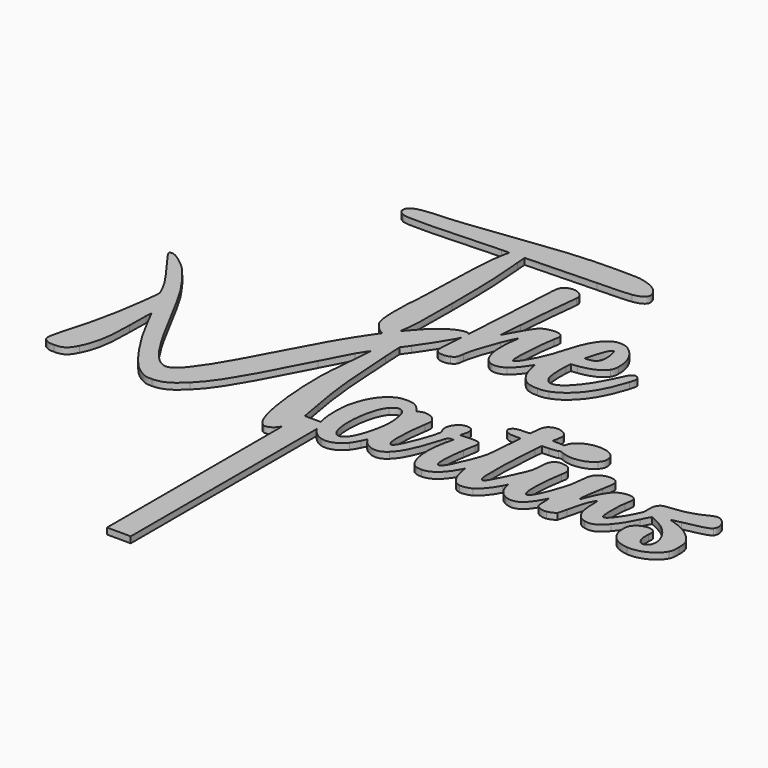
from build123d import *

# Parameters (mm, degrees)
F1_DEPTH = 1.524


# Not quite as in the source:
# - ends of sketch curves that miss each other by under 0.0002 mm in the source are joined


with BuildPart() as f1:
    # F0 (on Top) → F1 (new body)
    with BuildSketch(Plane.XY):
        with BuildLine():
            add(Edge.make_bspline(
                [(-16.4951387862, 3474.825739188), (-16.6800585023, 3474.8804924692), (-16.8650518694, 3474.9520282822), (-17.0115018566, 3475.0294197741)],
                knots=[0.5346499123, 0.5346499123, 0.5346499123, 0.5346499123, 1, 1, 1, 1], degree=3))
            add(Edge.make_bspline(
                [(-16.4951387862, 3474.825739188), (-15.7866961372, 3475.8123794255), (-15.094304248, 3476.7288703178), (-14.4178850512, 3477.5752871703)],
                knots=[0.0597909067, 0.0597909067, 0.0597909067, 0.0597909067, 0.2184884646, 0.2184884646, 0.2184884646, 0.2184884646], degree=3))
            add(Edge.make_bspline(
                [(-14.4058442585, 3477.6385135946), (-14.4097287654, 3477.6176536184), (-14.4137442865, 3477.5965715564), (-14.4178850512, 3477.5752871703)],
                knots=[0, 0, 0, 0, 0.0299805495, 0.0299805495, 0.0299805495, 0.0299805495], degree=3))
            add(Edge.make_bspline(
                [(-13.764209968, 3492.7401815257), (-13.7508003194, 3482.6742635991), (-13.8343750054, 3480.7073148376), (-14.4058442585, 3477.6385135946)],
                knots=[0, 0, 0, 0, 1, 1, 1, 1], degree=3))
            add(Edge.make_bspline(
                [(-14.5580975351, 3513.8236564948), (-13.9877605118, 3508.4516247626), (-13.7777050082, 3502.8731476952), (-13.764209968, 3492.7401815257)],
                knots=[0, 0, 0, 0, 1, 1, 1, 1], degree=3))
            add(Edge.make_bspline(
                [(-14.7308827548, 3516.2445566504), (-14.7727673494, 3516.2026736371), (-14.6950135262, 3515.1132677764), (-14.5580975351, 3513.8236564948)],
                knots=[0, 0, 0, 0, 1, 1, 1, 1], degree=3))
            add(Edge.make_bspline(
                [(2.5366157885, 3516.7758823493), (-6.7649300297, 3516.5842746005), (-14.6332769589, 3516.3421640277), (-14.7308827548, 3516.2445566504)],
                knots=[0, 0, 0, 0, 1, 1, 1, 1], degree=3))
            add(Edge.make_bspline(
                [(10.9317057324, 3517.1545373014), (10.1299399967, 3516.9908842422), (7.7392827101, 3516.8830551705), (2.5366157885, 3516.7758823493)],
                knots=[0, 0, 0, 0, 1, 1, 1, 1], degree=3))
            add(Edge.make_bspline(
                [(13.5480783988, 3520.1762023646), (14.3093700831, 3518.5046279958), (13.614522575, 3517.7021443379), (10.9317057324, 3517.1545373014)],
                knots=[0, 0, 0, 0, 1, 1, 1, 1], degree=3))
            add(Edge.make_bspline(
                [(8.6247227555, 3523.207953128), (11.0429694452, 3522.689428267), (12.9337378033, 3521.525111808), (13.5480783988, 3520.1762023646)],
                knots=[0, 0, 0, 0, 1, 1, 1, 1], degree=3))
            add(Edge.make_bspline(
                [(2.062217843, 3523.496576838), (6.5131268977, 3523.4962605727), (7.4782768672, 3523.4537782367), (8.6247227555, 3523.207953128)],
                knots=[0, 0, 0, 0, 1, 1, 1, 1], degree=3))
            add(Edge.make_bspline(
                [(-23.2390059159, 3521.3613464746), (-10.9639432633, 3523.0044806865), (-5.1261808362, 3523.4971429529), (2.062217843, 3523.496576838)],
                knots=[0, 0, 0, 0, 1, 1, 1, 1], degree=3))
            add(Edge.make_bspline(
                [(-37.4580975839, 3519.7783675035), (-36.0309520126, 3519.7811664514), (-30.1663086165, 3520.4340597865), (-23.2390059159, 3521.3613464746)],
                knots=[0, 0, 0, 0, 1, 1, 1, 1], degree=3))
            add(Edge.make_bspline(
                [(-43.4768191074, 3519.1378195843), (-42.3460378392, 3519.487082421), (-39.6493843899, 3519.7740757834), (-37.4580975839, 3519.7783675035)],
                knots=[0, 0, 0, 0, 1, 1, 1, 1], degree=3))
            add(Edge.make_bspline(
                [(-45.4566430292, 3517.290477614), (-45.4566430292, 3518.1528603379), (-44.8583655482, 3518.7111033763), (-43.4768191074, 3519.1378195843)],
                knots=[0, 0, 0, 0, 1, 1, 1, 1], degree=3))
            add(Edge.make_bspline(
                [(-44.1915818412, 3515.7274518205), (-45.1570717959, 3516.2424645554), (-45.4566430292, 3516.6125961578), (-45.4566430292, 3517.290477614)],
                knots=[0, 0, 0, 0, 1, 1, 1, 1], degree=3))
            add(Edge.make_bspline(
                [(-20.2740187566, 3516.06545245), (-37.5407345433, 3515.2545118581), (-43.1561956746, 3515.1751545697), (-44.1915818412, 3515.7274518205)],
                knots=[0, 0, 0, 0, 1, 1, 1, 1], degree=3))
            add(Edge.make_bspline(
                [(-18.4159601368, 3516.0222648424), (-18.4159601368, 3516.094014369), (-19.2520865158, 3516.1134488715), (-20.2740187566, 3516.06545245)],
                knots=[0, 0, 0, 0, 1, 1, 1, 1], degree=3))
            add(Edge.make_bspline(
                [(-18.7238728673, 3514.4760232482), (-18.5545207074, 3515.2547079426), (-18.4159601368, 3515.9505168971), (-18.4159601368, 3516.0222648424)],
                knots=[0, 0, 0, 0, 1, 1, 1, 1], degree=3))
            add(Edge.make_bspline(
                [(-19.8305136054, 3497.1663617968), (-19.6046068851, 3507.2168934167), (-19.3139859597, 3511.7626535966), (-18.7238728673, 3514.4760232482)],
                knots=[0, 0, 0, 0, 1, 1, 1, 1], degree=3))
            add(Edge.make_bspline(
                [(-20.0594944244, 3490.3666579116), (-20.0147033517, 3490.4962634303), (-19.9116625366, 3493.5561301787), (-19.8305136054, 3497.1663617968)],
                knots=[0, 0, 0, 0, 1, 1, 1, 1], degree=3))
            add(Edge.make_bspline(
                [(-20.3144422056, 3486.8892735315), (-20.2190123149, 3488.6722191432), (-20.1042870784, 3490.2370365797), (-20.0594944244, 3490.3666579116)],
                knots=[0, 0, 0, 0, 1, 1, 1, 1], degree=3))
            add(Edge.make_bspline(
                [(-19.8302368732, 3478.1253882061), (-20.3470112059, 3479.5065820111), (-20.5311772323, 3482.8399075484), (-20.3144422056, 3486.8892735315)],
                knots=[0, 0, 0, 0, 1, 1, 1, 1], degree=3))
            add(Edge.make_bspline(
                [(-17.0115018566, 3475.0294197741), (-18.0581945076, 3475.5825677785), (-19.4513605354, 3477.1127383516), (-19.8302368732, 3478.1253882061)],
                knots=[0, 0, 0, 0, 1, 1, 1, 1], degree=3))
        make_face()
        with BuildLine():
            Line((-56.2574582039, 3453.6457123253), (-54.4877957346, 3450.1823891003))
            add(Edge.make_bspline(
                [(-48.7301844216, 3440.3937599355), (-50.9593487409, 3443.67603551), (-52.5123046474, 3446.3162466731), (-54.4877957346, 3450.1823891003)],
                knots=[0, 0, 0, 0, 1, 1, 1, 1], degree=3))
            add(Edge.make_bspline(
                [(-41.7754741704, 3432.9327184318), (-43.9459380692, 3434.0343890607), (-45.6602446236, 3435.8735049705), (-48.7301844216, 3440.3937599355)],
                knots=[0, 0, 0, 0, 1, 1, 1, 1], degree=3))
            add(Edge.make_bspline(
                [(-39.1483073695, 3432.3396798854), (-40.5110945342, 3432.3295435827), (-40.6480516397, 3432.3604680034), (-41.7754741704, 3432.9327184318)],
                knots=[0, 0, 0, 0, 1, 1, 1, 1], degree=3))
            add(Edge.make_bspline(
                [(-32.502838163, 3435.8000523553), (-35.077889187, 3433.233766624), (-36.7608649197, 3432.3574207873), (-39.1483073695, 3432.3396798854)],
                knots=[0, 0, 0, 0, 1, 1, 1, 1], degree=3))
            add(Edge.make_bspline(
                [(-18.9330217551, 3458.1046165667), (-26.3784697984, 3443.5673335461), (-28.94959597, 3439.3412005633), (-32.502838163, 3435.8000523553)],
                knots=[0, 0, 0, 0, 1, 1, 1, 1], degree=3))
            add(Edge.make_bspline(
                [(-15.3817451509, 3464.910389583), (-15.6422655267, 3464.4721866194), (-17.2403414217, 3461.4095889202), (-18.9330217551, 3458.1046165667)],
                knots=[0, 0, 0, 0, 1, 1, 1, 1], degree=3))
            add(Edge.make_bspline(
                [(-13.6368019773, 3467.5135091521), (-13.722075008, 3467.5135091521), (-14.7129752979, 3466.0352772473), (-15.3817451509, 3464.910389583)],
                knots=[0, 0, 0, 0, 1, 1, 1, 1], degree=3))
            add(Edge.make_bspline(
                [(-14.1663692412, 3460.3975399699), (-13.7542202128, 3464.3164749818), (-13.5162985738, 3467.5135091521), (-13.6368019773, 3467.5135091521)],
                knots=[0, 0, 0, 0, 1, 1, 1, 1], degree=3))
            add(Edge.make_bspline(
                [(-14.5609813588, 3447.9841270632), (-14.7854601413, 3452.0795128096), (-14.6746866397, 3455.5641855235), (-14.1663692412, 3460.3975399699)],
                knots=[0, 0, 0, 0, 1, 1, 1, 1], degree=3))
            add(Edge.make_bspline(
                [(-11.0901911101, 3431.1923010145), (-12.8122066311, 3432.9143165355), (-14.0679759446, 3438.9897792159), (-14.5609813588, 3447.9841270632)],
                knots=[0, 0, 0, 0, 1, 1, 1, 1], degree=3))
            add(Edge.make_bspline(
                [(-10.2336814328, 3430.6335930661), (-10.4286321059, 3430.6647531045), (-10.8140614606, 3430.916171365), (-11.0901911101, 3431.1923010145)],
                knots=[0, 0, 0, 0, 1, 1, 1, 1], degree=3))
            add(Edge.make_bspline(
                [(-7.840324822, 3431.8184825826), (-8.489377115, 3430.9675296866), (-9.4249847431, 3430.5043354393), (-10.2336814328, 3430.6335930661)],
                knots=[0, 0, 0, 0, 1, 1, 1, 1], degree=3))
            add(Edge.make_bspline(
                [(-7.3343984416, 3432.5808147994), (-7.4816183586, 3432.321105511), (-7.6498403129, 3432.0682205632), (-7.840324822, 3431.8184825826)],
                knots=[0.7774513502, 0.7774513502, 0.7774513502, 0.7774513502, 1, 1, 1, 1], degree=3))
            Line((-7.3343984416, 3432.5808147994), (-7.3343984416, 3438.6502356796))
            Line((-7.3343984416, 3438.6502356796), (-6.6488588735, 3438.6502356796))
            add(Edge.make_bspline(
                [(-7.5903503126, 3443.9517445266), (-7.1005108992, 3441.4777591259), (-6.8078684627, 3439.8717466959), (-6.6488588735, 3438.6502356796)],
                knots=[0, 0, 0, 0, 0.5048196065, 0.5048196065, 0.5048196065, 0.5048196065], degree=3))
            add(Edge.make_bspline(
                [(-10.0368094481, 3467.7243205298), (-9.4481780587, 3456.3496999669), (-8.8021318672, 3450.0719824664), (-7.5903503126, 3443.9517445266)],
                knots=[0, 0, 0, 0, 1, 1, 1, 1], degree=3))
            Line((-10.0368094481, 3467.7243205298), (-10.2727591729, 3472.2837781597))
            Line((-10.2727591729, 3472.2837781597), (-8.8698205474, 3474.2172534022))
            add(Edge.make_bspline(
                [(-3.8857119219, 3482.0310698688), (-4.5791504681, 3480.6626342059), (-7.3860524187, 3476.2621251889), (-8.8698205474, 3474.2172534022)],
                knots=[0, 0, 0, 0, 1, 1, 1, 1], degree=3))
            add(Edge.make_bspline(
                [(-3.5395519409, 3482.8531070297), (-3.6464231613, 3482.5565940157), (-3.7706794884, 3482.2580737216), (-3.8857119219, 3482.0310698688)],
                knots=[0.4932655399, 0.4932655399, 0.4932655399, 0.4932655399, 1, 1, 1, 1], degree=3))
            add(Edge.make_bspline(
                [(-3.5395519361, 3482.8531070287), (-3.4918571938, 3483.5093905716), (-3.4436011891, 3484.1852250498), (-3.3951575292, 3484.8747923712)],
                knots=[0.121112451, 0.121112451, 0.121112451, 0.121112451, 0.2158785304, 0.2158785304, 0.2158785304, 0.2158785304], degree=3))
            add(Edge.make_bspline(
                [(-5.5774766672, 3484.9908022801), (-4.4187556834, 3485.3423771205), (-3.6978778733, 3485.3075858697), (-3.3951575098, 3484.8747923775)],
                knots=[0, 0, 0, 0, 0.6224653627, 0.6224653627, 0.6224653627, 0.6224653627], degree=3))
            add(Edge.make_bspline(
                [(-14.4178850512, 3477.5752871703), (-11.0868356496, 3481.7434958245), (-8.1431405884, 3484.2123364092), (-5.5774766672, 3484.9908022801)],
                knots=[0.2184884646, 0.2184884646, 0.2184884646, 0.2184884646, 1, 1, 1, 1], degree=3))
            add(Edge.make_bspline(
                [(-14.4178850512, 3477.5752871703), (-14.5518593236, 3476.8866317296), (-14.8169440207, 3475.9861746652), (-15.0176831954, 3475.5432560021)],
                knots=[0.0299805495, 0.0299805495, 0.0299805495, 0.0299805495, 1, 1, 1, 1], degree=3))
            add(Edge.make_bspline(
                [(-15.0176831954, 3475.5432560021), (-15.3628867671, 3474.7815942874), (-15.4370841871, 3474.7136446883), (-15.916623025, 3474.7200490606)],
                knots=[0, 0, 0, 0, 1, 1, 1, 1], degree=3))
            add(Edge.make_bspline(
                [(-15.916623025, 3474.7200490606), (-16.0703201742, 3474.7220781551), (-16.2826808699, 3474.7628320611), (-16.4951387862, 3474.825739188)],
                knots=[0, 0, 0, 0, 0.5346499123, 0.5346499123, 0.5346499123, 0.5346499123], degree=3))
            add(Edge.make_bspline(
                [(-17.3027168449, 3473.6806824433), (-17.0312429994, 3474.0723282808), (-16.7620517048, 3474.4540125199), (-16.4951387862, 3474.825739188)],
                knots=[0, 0, 0, 0, 0.0597909067, 0.0597909067, 0.0597909067, 0.0597909067], degree=3))
            add(Edge.make_bspline(
                [(-27.1440658534, 3456.8697112749), (-22.5396368796, 3465.6083143524), (-20.5916703611, 3468.9358253523), (-17.3027168449, 3473.6806824433)],
                knots=[0, 0, 0, 0, 1, 1, 1, 1], degree=3))
            add(Edge.make_bspline(
                [(-36.4910811334, 3441.0044792933), (-34.0927812959, 3444.0904363473), (-32.0556058252, 3447.5482518122), (-27.1440658534, 3456.8697112749)],
                knots=[0, 0, 0, 0, 1, 1, 1, 1], degree=3))
            add(Edge.make_bspline(
                [(-40.369586371, 3438.1043091253), (-39.1970723156, 3438.096228547), (-38.1327937328, 3438.8920437511), (-36.4910811334, 3441.0044792933)],
                knots=[0, 0, 0, 0, 1, 1, 1, 1], degree=3))
            add(Edge.make_bspline(
                [(-47.3935397464, 3445.5162630923), (-44.7686611249, 3440.8615732375), (-42.1674834247, 3438.116706725), (-40.369586371, 3438.1043091253)],
                knots=[0, 0, 0, 0, 1, 1, 1, 1], degree=3))
            add(Edge.make_bspline(
                [(-48.7851940261, 3447.9160256568), (-48.5890241503, 3447.6055891292), (-47.9627809104, 3446.5256965287), (-47.3935397464, 3445.5162630923)],
                knots=[0, 0, 0, 0, 1, 1, 1, 1], degree=3))
            add(Edge.make_bspline(
                [(-51.6322332055, 3453.2134693813), (-50.2625309, 3450.6103118604), (-48.9813623205, 3448.2264621843), (-48.7851940261, 3447.9160256568)],
                knots=[0, 0, 0, 0, 1, 1, 1, 1], degree=3))
            add(Edge.make_bspline(
                [(-57.8490759616, 3464.4830187058), (-56.3952502498, 3462.1380902186), (-54.9414213754, 3459.5026688934), (-51.6322332055, 3453.2134693813)],
                knots=[0, 0, 0, 0, 1, 1, 1, 1], degree=3))
            add(Edge.make_bspline(
                [(-63.0135538486, 3471.4352652504), (-61.5574700026, 3469.8649811683), (-59.3104436124, 3466.8401107564), (-57.8490759616, 3464.4830187058)],
                knots=[0, 0, 0, 0, 1, 1, 1, 1], degree=3))
            add(Edge.make_bspline(
                [(-68.7254664075, 3475.5782742252), (-67.7419287737, 3475.5782742252), (-65.0339055869, 3473.6140706465), (-63.0135538486, 3471.4352652504)],
                knots=[0, 0, 0, 0, 1, 1, 1, 1], degree=3))
            add(Edge.make_bspline(
                [(-66.2668437086, 3470.7744431443), (-69.7205508873, 3475.3821802531), (-69.8209129353, 3475.5782742252), (-68.7254664075, 3475.5782742252)],
                knots=[0, 0, 0, 0, 1, 1, 1, 1], degree=3))
            add(Edge.make_bspline(
                [(-60.9473141901, 3462.7309152858), (-61.9172707991, 3464.737201125), (-63.2340208058, 3466.7282271636), (-66.2668437086, 3470.7744431443)],
                knots=[0, 0, 0, 0, 1, 1, 1, 1], degree=3))
            add(Edge.make_bspline(
                [(-60.330889604, 3459.7650093759), (-60.1653972644, 3461.0192163389), (-60.1997966501, 3461.1847274567), (-60.9473141901, 3462.7309152858)],
                knots=[0, 0, 0, 0, 1, 1, 1, 1], degree=3))
            add(Edge.make_bspline(
                [(-60.7262975243, 3456.4219918885), (-60.5604653971, 3457.86927249), (-60.3825319714, 3459.3736310709), (-60.330889604, 3459.7650093759)],
                knots=[0, 0, 0, 0, 1, 1, 1, 1], degree=3))
            add(Edge.make_bspline(
                [(-64.6322818676, 3437.7794682948), (-62.743153345, 3444.1123551137), (-61.4048953214, 3450.4996063558), (-60.7262975243, 3456.4219918885)],
                knots=[0, 0, 0, 0, 1, 1, 1, 1], degree=3))
            add(Edge.make_bspline(
                [(-65.4686612587, 3434.4119339216), (-65.3597394904, 3435.0871366108), (-64.9833695551, 3436.6025265252), (-64.6322818676, 3437.7794682948)],
                knots=[0, 0, 0, 0, 1, 1, 1, 1], degree=3))
            add(Edge.make_bspline(
                [(-64.6167247776, 3432.0724293842), (-65.5929930536, 3432.6318299535), (-65.7058349302, 3432.9417051102), (-65.4686612587, 3434.4119339216)],
                knots=[0, 0, 0, 0, 1, 1, 1, 1], degree=3))
            add(Edge.make_bspline(
                [(-62.616462211, 3431.6983618602), (-63.7444982964, 3431.6967647204), (-64.066075269, 3431.7569073106), (-64.6167247776, 3432.0724293842)],
                knots=[0, 0, 0, 0, 1, 1, 1, 1], degree=3))
            add(Edge.make_bspline(
                [(-58.5744363502, 3434.4829354808), (-59.6836665104, 3432.2802979133), (-60.5241049689, 3431.7013157781), (-62.616462211, 3431.6983618602)],
                knots=[0, 0, 0, 0, 1, 1, 1, 1], degree=3))
            add(Edge.make_bspline(
                [(-56.4171073445, 3447.0353311722), (-56.3913222348, 3441.1183553574), (-56.9915006679, 3437.6262251078), (-58.5744363502, 3434.4829354808)],
                knots=[0, 0, 0, 0, 1, 1, 1, 1], degree=3))
            add(Edge.make_bspline(
                [(-56.3445197148, 3452.000914558), (-56.3924022808, 3451.0962756278), (-56.425067742, 3448.8617632623), (-56.4171073445, 3447.0353311722)],
                knots=[0, 0, 0, 0, 1, 1, 1, 1], degree=3))
            Line((-56.3445197148, 3452.000914558), (-56.2574582039, 3453.6457123253))
        make_face()
        with BuildLine():
            add(Edge.make_bspline(
                [(-3.301422855, 3483.6454808665), (-3.3479639421, 3483.4284685297), (-3.4355213403, 3483.1417387756), (-3.5395519409, 3482.8531070297)],
                knots=[0, 0, 0, 0, 0.4932655399, 0.4932655399, 0.4932655399, 0.4932655399], degree=3))
            add(Edge.make_bspline(
                [(-3.7188856562, 3480.4448304544), (-3.660544386, 3481.2075598501), (-3.6005065222, 3482.0143669549), (-3.5395519409, 3482.8531070297)],
                knots=[0, 0, 0, 0, 0.121112451, 0.121112451, 0.121112451, 0.121112451], degree=3))
            add(Edge.make_bspline(
                [(-3.1856006938, 3475.3377309988), (-4.0624019525, 3475.8723458569), (-4.0659994703, 3475.906802961), (-3.7188856562, 3480.4448304544)],
                knots=[0, 0, 0, 0, 1, 1, 1, 1], degree=3))
            add(Edge.make_bspline(
                [(-0.2639387175, 3475.3287648777), (-1.0620152186, 3474.9214468017), (-2.5101702936, 3474.9258903291), (-3.1856006938, 3475.3377309988)],
                knots=[0, 0, 0, 0, 1, 1, 1, 1], degree=3))
            add(Edge.make_bspline(
                [(1.0625617483, 3477.6703456968), (0.8960101176, 3476.1384356645), (0.7225623221, 3475.8322592305), (-0.2639387175, 3475.3287648777)],
                knots=[0, 0, 0, 0, 1, 1, 1, 1], degree=3))
            add(Edge.make_bspline(
                [(3.5972320192, 3485.9404776405), (2.2704516585, 3482.5973320657), (1.2286753516, 3479.1982233465), (1.0625617483, 3477.6703456968)],
                knots=[0, 0, 0, 0, 1, 1, 1, 1], degree=3))
            add(Edge.make_bspline(
                [(5.2550361969, 3489.3628792988), (5.1405260208, 3489.4773989628), (4.3679057135, 3487.8823781905), (3.5972320192, 3485.9404776405)],
                knots=[0, 0, 0, 0, 1, 1, 1, 1], degree=3))
            add(Edge.make_bspline(
                [(5.0713414058, 3487.9181794221), (5.2043325445, 3488.680805746), (5.2869948052, 3489.3309206905), (5.2550361969, 3489.3628792988)],
                knots=[0, 0, 0, 0, 1, 1, 1, 1], degree=3))
            add(Edge.make_bspline(
                [(4.983539834, 3482.1273460211), (4.7530709868, 3483.4020691138), (4.7977576919, 3486.3493454164), (5.0713414058, 3487.9181794221)],
                knots=[0, 0, 0, 0, 1, 1, 1, 1], degree=3))
            add(Edge.make_bspline(
                [(7.6110814093, 3477.9409422849), (6.2673666234, 3478.4541143558), (5.3969112278, 3479.8410009361), (4.983539834, 3482.1273460211)],
                knots=[0, 0, 0, 0, 1, 1, 1, 1], degree=3))
            add(Edge.make_bspline(
                [(11.0315064095, 3478.5305714913), (9.9027539832, 3477.8062607081), (8.5667940223, 3477.5759563189), (7.6110814093, 3477.9409422849)],
                knots=[0, 0, 0, 0, 1, 1, 1, 1], degree=3))
            add(Edge.make_bspline(
                [(14.1259899759, 3482.1316788556), (13.3519701947, 3480.814212508), (11.8298153655, 3479.0428422061), (11.0315064095, 3478.5305714913)],
                knots=[0, 0, 0, 0, 1, 1, 1, 1], degree=3))
            Line((14.1259899759, 3482.1316788556), (14.5360516534, 3482.8296447396))
            Line((14.5360516534, 3482.8296447396), (14.8073092359, 3481.5782145859))
            add(Edge.make_bspline(
                [(16.4588181529, 3477.5675278487), (15.662568084, 3478.6491709777), (15.1972738351, 3479.7791236307), (14.8073092359, 3481.5782145859)],
                knots=[0, 0, 0, 0, 1, 1, 1, 1], degree=3))
            add(Edge.make_bspline(
                [(21.0381356622, 3475.4371964347), (18.8022839132, 3475.4327687206), (17.6283023868, 3475.9788956354), (16.4588181529, 3477.5675278487)],
                knots=[0, 0, 0, 0, 1, 1, 1, 1], degree=3))
            add(Edge.make_bspline(
                [(23.5682580381, 3475.8376989936), (22.6999658971, 3475.5257507179), (22.154511046, 3475.4394102918), (21.0381356622, 3475.4371964347)],
                knots=[0, 0, 0, 0, 1, 1, 1, 1], degree=3))
            add(Edge.make_bspline(
                [(33.1572652914, 3488.5029855828), (31.1569584476, 3481.8590265431), (27.7301796776, 3477.3329064381), (23.5682580381, 3475.8376989936)],
                knots=[0, 0, 0, 0, 1, 1, 1, 1], degree=3))
            add(Edge.make_bspline(
                [(32.8994885171, 3491.1109724748), (33.651032905, 3490.7525806403), (33.6963916739, 3490.2936638811), (33.1572652914, 3488.5029855828)],
                knots=[0, 0, 0, 0, 1, 1, 1, 1], degree=3))
            add(Edge.make_bspline(
                [(31.9313624912, 3491.1365108975), (32.3257010394, 3491.3252264003), (32.4574777193, 3491.321747482), (32.8994885171, 3491.1109724748)],
                knots=[0, 0, 0, 0, 1, 1, 1, 1], degree=3))
            add(Edge.make_bspline(
                [(31.2100261831, 3490.3664048994), (31.3557011416, 3490.669814012), (31.6803031918, 3491.0163775245), (31.9313624912, 3491.1365108975)],
                knots=[0, 0, 0, 0, 1, 1, 1, 1], degree=3))
            add(Edge.make_bspline(
                [(29.8435988048, 3487.5218041254), (30.449457165, 3488.7829119972), (31.0643496434, 3490.0629799735), (31.2100261831, 3490.3664048994)],
                knots=[0, 0, 0, 0, 1, 1, 1, 1], degree=3))
            add(Edge.make_bspline(
                [(25.2460517639, 3480.5527718002), (26.7766540392, 3482.0754943256), (28.4340344214, 3484.5877793388), (29.8435988048, 3487.5218041254)],
                knots=[0, 0, 0, 0, 1, 1, 1, 1], degree=3))
            add(Edge.make_bspline(
                [(21.9211926485, 3478.6663758098), (22.9317820345, 3478.6663758098), (23.9048180792, 3479.2184485122), (25.2460517639, 3480.5527718002)],
                knots=[0, 0, 0, 0, 1, 1, 1, 1], degree=3))
            add(Edge.make_bspline(
                [(19.9306331012, 3480.5723011823), (20.3094635806, 3479.3572099113), (21.0309675092, 3478.6663758098), (21.9211926485, 3478.6663758098)],
                knots=[0, 0, 0, 0, 1, 1, 1, 1], degree=3))
            add(Edge.make_bspline(
                [(19.6069687776, 3485.9779392649), (19.4547661034, 3484.1507797647), (19.6068454341, 3481.6108531646), (19.9306331012, 3480.5723011823)],
                knots=[0, 0, 0, 0, 1, 1, 1, 1], degree=3))
            Line((19.6069687776, 3485.9779392649), (19.7181075656, 3487.3121676733))
            Line((19.7181075656, 3487.3121676733), (21.2162325575, 3487.5081572779))
            add(Edge.make_bspline(
                [(27.0846142094, 3490.238254201), (26.1960020232, 3488.8955024429), (23.9954865958, 3487.8717833031), (21.2162325575, 3487.5081572779)],
                knots=[0, 0, 0, 0, 1, 1, 1, 1], degree=3))
            add(Edge.make_bspline(
                [(27.5768590056, 3492.113754852), (27.5310527213, 3491.1068768392), (27.4466620708, 3490.7853299118), (27.0846142094, 3490.238254201)],
                knots=[0, 0, 0, 0, 1, 1, 1, 1], degree=3))
            add(Edge.make_bspline(
                [(25.0059494757, 3498.5539916006), (26.7593021436, 3496.9138081439), (27.6892486229, 3494.5842612194), (27.5768590056, 3492.113754852)],
                knots=[0, 0, 0, 0, 1, 1, 1, 1], degree=3))
            add(Edge.make_bspline(
                [(21.6820296683, 3500.0108202514), (22.9531331047, 3500.0163548941), (23.8743142913, 3499.6125789894), (25.0059494757, 3498.5539916006)],
                knots=[0, 0, 0, 0, 1, 1, 1, 1], degree=3))
            add(Edge.make_bspline(
                [(15.1826845169, 3491.237921365), (16.6399654271, 3496.8318479922), (18.9864388703, 3499.9991500619), (21.6820296683, 3500.0108202514)],
                knots=[0, 0, 0, 0, 1, 1, 1, 1], degree=3))
            add(Edge.make_bspline(
                [(11.5406682364, 3482.749424047), (13.07443949, 3485.1272804956), (14.3889060613, 3488.1909266143), (15.1826845169, 3491.237921365)],
                knots=[0, 0, 0, 0, 1, 1, 1, 1], degree=3))
            add(Edge.make_bspline(
                [(10.0721425137, 3481.5517906203), (10.3716742138, 3481.2522715708), (10.8005979535, 3481.6020609893), (11.5406682364, 3482.749424047)],
                knots=[0, 0, 0, 0, 1, 1, 1, 1], degree=3))
            add(Edge.make_bspline(
                [(10.7689540292, 3493.3322934147), (10.0735309183, 3490.1320523143), (9.5942767192, 3482.0296674841), (10.0721425137, 3481.5517906203)],
                knots=[0, 0, 0, 0, 1, 1, 1, 1], degree=3))
            add(Edge.make_bspline(
                [(10.4849066781, 3495.6397650215), (11.0271419484, 3495.2367165271), (11.0834276833, 3494.7794601607), (10.7689540292, 3493.3322934147)],
                knots=[0, 0, 0, 0, 1, 1, 1, 1], degree=3))
            add(Edge.make_bspline(
                [(5.9370132887, 3495.1916487222), (7.1459864076, 3496.0835959261), (9.5668834005, 3496.3221390263), (10.4849066781, 3495.6397650215)],
                knots=[0, 0, 0, 0, 1, 1, 1, 1], degree=3))
            add(Edge.make_bspline(
                [(2.4248175873, 3489.8147275286), (4.1401156334, 3493.0214678808), (5.2048101051, 3494.6514359685), (5.9370132887, 3495.1916487222)],
                knots=[0, 0, 0, 0, 1, 1, 1, 1], degree=3))
            Line((2.4248175873, 3489.8147275286), (1.6635464602, 3488.3915336921))
            Line((1.6635464602, 3488.3915336921), (1.7489728796, 3489.4193959074))
            add(Edge.make_bspline(
                [(2.0702256803, 3493.9261763894), (1.9405221194, 3492.0127713426), (1.7959572521, 3489.9847201257), (1.7489728796, 3489.4193959074)],
                knots=[0, 0, 0, 0, 1, 1, 1, 1], degree=3))
            add(Edge.make_bspline(
                [(3.5023729873, 3509.3441096175), (3.0602325208, 3505.8495520317), (2.3876390203, 3498.6086738705), (2.0702256803, 3493.9261763894)],
                knots=[0, 0, 0, 0, 1, 1, 1, 1], degree=3))
            add(Edge.make_bspline(
                [(2.146034472, 3511.5184335343), (3.1461823592, 3511.0131839091), (3.6178746551, 3510.2570252105), (3.5023729873, 3509.3441096175)],
                knots=[0, 0, 0, 0, 1, 1, 1, 1], degree=3))
            add(Edge.make_bspline(
                [(-1.5014105023, 3510.7593810082), (-0.7438665617, 3511.8232500275), (0.8755524969, 3512.160262328), (2.146034472, 3511.5184335343)],
                knots=[0, 0, 0, 0, 1, 1, 1, 1], degree=3))
            add(Edge.make_bspline(
                [(-2.365749327, 3501.5165435171), (-1.9443969785, 3509.9288208985), (-1.9219563743, 3510.1687871926), (-1.5014105023, 3510.7593810082)],
                knots=[0, 0, 0, 0, 1, 1, 1, 1], degree=3))
            add(Edge.make_bspline(
                [(-3.3951575292, 3484.8747923712), (-2.9943209219, 3490.5804683344), (-2.5806367367, 3497.2263466322), (-2.365749327, 3501.5165435171)],
                knots=[0.2158785304, 0.2158785304, 0.2158785304, 0.2158785304, 1, 1, 1, 1], degree=3))
            add(Edge.make_bspline(
                [(-3.3951575292, 3484.8747923712), (-3.2115530404, 3484.6122965925), (-3.1817722025, 3484.2033914808), (-3.301422855, 3483.6454808665)],
                knots=[0.6224653627, 0.6224653627, 0.6224653627, 0.6224653627, 1, 1, 1, 1], degree=3))
        make_face()
        with BuildLine():
            Line((20.3089528121, 3490.7965415165), (20.4186873822, 3491.2544304135))
            add(Edge.make_bspline(
                [(22.7127572471, 3496.693497738), (22.1171949037, 3496.693497738), (21.202353255, 3494.5244870782), (20.4186873822, 3491.2544304135)],
                knots=[0, 0, 0, 0, 1, 1, 1, 1], degree=3))
            add(Edge.make_bspline(
                [(23.4422437118, 3494.0843090379), (23.3757805596, 3495.4751173079), (23.0351422775, 3496.693497738), (22.7127572471, 3496.693497738)],
                knots=[0, 0, 0, 0, 1, 1, 1, 1], degree=3))
            add(Edge.make_bspline(
                [(22.5310928792, 3491.2803957944), (23.3023991041, 3491.8451507352), (23.5176002441, 3492.5074102671), (23.4422437118, 3494.0843090379)],
                knots=[0, 0, 0, 0, 1, 1, 1, 1], degree=3))
            add(Edge.make_bspline(
                [(21.2177047725, 3490.8903299904), (21.7237972447, 3490.9425612042), (22.3057491111, 3491.115400189), (22.5310928792, 3491.2803957944)],
                knots=[0, 0, 0, 0, 1, 1, 1, 1], degree=3))
            Line((21.2177047725, 3490.8903299904), (20.3089528121, 3490.7965415166))
        make_face(mode=Mode.SUBTRACT)
        with BuildLine():
            add(Edge.make_bspline(
                [(-2.7065495837, 3438.6502356796), (-2.8504175737, 3439.1276985239), (-2.9741278396, 3439.6305412044), (-3.0761628972, 3440.1565609628)],
                knots=[0.8554130144, 0.8554130144, 0.8554130144, 0.8554130144, 1, 1, 1, 1], degree=3))
            Line((-2.7065495837, 3438.6502356796), (-1.5014105023, 3438.6502356796))
            Line((-1.5014105023, 3438.6502356796), (-1.5014105023, 3435.9241050302))
            add(Edge.make_bspline(
                [(1.6493703841, 3433.2970513099), (0.4155031896, 3433.6719856025), (-0.6613738199, 3434.5863066193), (-1.5014105023, 3435.9241050302)],
                knots=[0, 0, 0, 0, 0.541809208, 0.541809208, 0.541809208, 0.541809208], degree=3))
            add(Edge.make_bspline(
                [(6.9959032267, 3435.3335151837), (5.6751999037, 3433.5817659809), (3.4729181347, 3432.7429292084), (1.6493703841, 3433.2970513099)],
                knots=[0, 0, 0, 0, 1, 1, 1, 1], degree=3))
            add(Edge.make_bspline(
                [(8.1880874023, 3437.3475779866), (7.8602452141, 3436.674707754), (7.3237612281, 3435.7683799671), (6.9959032267, 3435.3335151837)],
                knots=[0, 0, 0, 0, 1, 1, 1, 1], degree=3))
            Line((8.1880874023, 3437.3475779866), (8.7841668394, 3438.5709791283))
            Line((8.7841668394, 3438.5709791283), (9.3357619812, 3437.8265016885))
            add(Edge.make_bspline(
                [(12.6735737419, 3436.045112102), (11.5588397749, 3436.045112102), (10.0648641836, 3436.8424469609), (9.3357619812, 3437.8265016885)],
                knots=[0, 0, 0, 0, 1, 1, 1, 1], degree=3))
            add(Edge.make_bspline(
                [(15.2801674852, 3437.1795146078), (14.3607225952, 3436.3374582545), (13.6889798483, 3436.045112102), (12.6735737419, 3436.045112102)],
                knots=[0, 0, 0, 0, 1, 1, 1, 1], degree=3))
            add(Edge.make_bspline(
                [(20.391356251, 3448.2207551771), (18.4978395475, 3441.8244729794), (17.1332148814, 3438.876597354), (15.2801674852, 3437.1795146078)],
                knots=[0, 0, 0, 0, 1, 1, 1, 1], degree=3))
            add(Edge.make_bspline(
                [(21.1277626005, 3448.7180127782), (20.648124139, 3448.6386602339), (20.4818286832, 3448.5263702402), (20.391356251, 3448.2207551771)],
                knots=[0, 0, 0, 0, 1, 1, 1, 1], degree=3))
            add(Edge.make_bspline(
                [(21.7705307021, 3448.7976499613), (21.7577535841, 3448.8102215069), (21.4685115754, 3448.7743870674), (21.1277626005, 3448.7180127782)],
                knots=[0, 0, 0, 0, 1, 1, 1, 1], degree=3))
            add(Edge.make_bspline(
                [(21.4969580576, 3447.612649752), (21.6601968093, 3448.2518266612), (21.7833030761, 3448.7850768344), (21.7705307021, 3448.7976499613)],
                knots=[0, 0, 0, 0, 1, 1, 1, 1], degree=3))
            add(Edge.make_bspline(
                [(21.7303349642, 3437.0307845265), (20.5224229154, 3439.4037467697), (20.4332392643, 3443.4475243449), (21.4969580576, 3447.612649752)],
                knots=[0, 0, 0, 0, 1, 1, 1, 1], degree=3))
            add(Edge.make_bspline(
                [(24.7225873547, 3435.2559938155), (23.1226723769, 3435.2534636931), (22.4241467034, 3435.6677823014), (21.7303349642, 3437.0307845265)],
                knots=[0, 0, 0, 0, 1, 1, 1, 1], degree=3))
            add(Edge.make_bspline(
                [(30.4508951066, 3439.8747780711), (28.8502226734, 3436.8789028616), (26.841610703, 3435.2593399023), (24.7225873547, 3435.2559938155)],
                knots=[0, 0, 0, 0, 1, 1, 1, 1], degree=3))
            Line((30.4508951066, 3439.8747780711), (30.9562902138, 3440.8206975292))
            Line((30.9562902138, 3440.8206975292), (31.1591158927, 3439.7374999563))
            add(Edge.make_bspline(
                [(34.4342834047, 3434.7035748025), (32.8112684096, 3435.0384807761), (31.7269133057, 3436.7051308942), (31.1591158927, 3439.7374999563)],
                knots=[0, 0, 0, 0, 1, 1, 1, 1], degree=3))
            add(Edge.make_bspline(
                [(37.3233716366, 3435.2953103359), (36.6150069497, 3434.879260175), (35.0933012173, 3434.5675886315), (34.4342834047, 3434.7035748025)],
                knots=[0, 0, 0, 0, 1, 1, 1, 1], degree=3))
            add(Edge.make_bspline(
                [(41.0288955701, 3439.7299190771), (40.0232541546, 3437.8005742594), (38.5144046065, 3435.994851221), (37.3233716366, 3435.2953103359)],
                knots=[0, 0, 0, 0, 1, 1, 1, 1], degree=3))
            Line((41.0288955701, 3439.7299190771), (41.5637349765, 3440.7560181133))
            Line((41.5637349765, 3440.7560181133), (41.7441058193, 3440.0397056795))
            add(Edge.make_bspline(
                [(44.3042575851, 3436.5329560665), (43.0131978085, 3437.1781056459), (42.1758632961, 3438.3250385827), (41.7441058193, 3440.0397056795)],
                knots=[0, 0, 0, 0, 1, 1, 1, 1], degree=3))
            add(Edge.make_bspline(
                [(50.8613559424, 3440.3146936113), (48.8429666303, 3436.4713887012), (46.7932085447, 3435.2892127409), (44.3042575851, 3436.5329560665)],
                knots=[0, 0, 0, 0, 1, 1, 1, 1], degree=3))
            Line((50.8613559424, 3440.3146936113), (51.3181110282, 3441.184423178))
            Line((51.3181110282, 3441.184423178), (51.3971773525, 3439.3911388537))
            add(Edge.make_bspline(
                [(51.9136306758, 3437.2222309801), (51.4945253922, 3437.5821535387), (51.4729387044, 3437.6728078234), (51.3971773525, 3439.3911388537)],
                knots=[0, 0, 0, 0, 1, 1, 1, 1], degree=3))
            add(Edge.make_bspline(
                [(54.3009070864, 3436.6066363928), (53.4867073805, 3436.4711040624), (52.4885519646, 3436.7284934117), (51.9136306758, 3437.2222309801)],
                knots=[0, 0, 0, 0, 1, 1, 1, 1], degree=3))
            add(Edge.make_bspline(
                [(56.2887072189, 3437.5346204459), (55.9854056365, 3437.1691648259), (55.0461688641, 3436.7306914555), (54.3009070864, 3436.6066363928)],
                knots=[0, 0, 0, 0, 1, 1, 1, 1], degree=3))
            add(Edge.make_bspline(
                [(56.8735323555, 3439.6913394549), (56.6648810698, 3438.6413038797), (56.4017088096, 3437.6707805628), (56.2887072189, 3437.5346204459)],
                knots=[0, 0, 0, 0, 1, 1, 1, 1], degree=3))
            add(Edge.make_bspline(
                [(59.1433525787, 3446.007468957), (58.6417241912, 3446.007468957), (57.4939658019, 3442.8136543674), (56.8735323555, 3439.6913394549)],
                knots=[0, 0, 0, 0, 1, 1, 1, 1], degree=3))
            add(Edge.make_bspline(
                [(59.3065549599, 3444.38660931), (59.3048787538, 3445.3756088455), (59.2412588267, 3446.007468957), (59.1433525787, 3446.007468957)],
                knots=[0, 0, 0, 0, 1, 1, 1, 1], degree=3))
            add(Edge.make_bspline(
                [(62.462912669, 3438.1016888673), (60.3742982291, 3438.6027384894), (59.3127727357, 3440.716445418), (59.3065549599, 3444.38660931)],
                knots=[0, 0, 0, 0, 1, 1, 1, 1], degree=3))
            add(Edge.make_bspline(
                [(67.2104437831, 3440.2389196088), (65.5503150555, 3438.2651458421), (64.2401449482, 3437.6753363645), (62.462912669, 3438.1016888673)],
                knots=[0, 0, 0, 0, 1, 1, 1, 1], degree=3))
            add(Edge.make_bspline(
                [(70.3456006481, 3445.2512770506), (69.1794925462, 3442.8543687805), (68.5099636565, 3441.7839562322), (67.2104437831, 3440.2389196088)],
                knots=[0, 0, 0, 0, 1, 1, 1, 1], degree=3))
            add(Edge.make_bspline(
                [(71.5635525387, 3447.4256009674), (71.4741269446, 3447.4228178328), (70.9260470916, 3446.4443720702), (70.3456006481, 3445.2512770506)],
                knots=[0, 0, 0, 0, 1, 1, 1, 1], degree=3))
            add(Edge.make_bspline(
                [(74.7680869405, 3445.8298527849), (73.9623378434, 3446.3707992742), (71.8276087605, 3447.4338207024), (71.5635525387, 3447.4256009674)],
                knots=[0, 0, 0, 0, 1, 1, 1, 1], degree=3))
            add(Edge.make_bspline(
                [(78.533631702, 3438.6698879373), (79.343569733, 3440.6083427769), (77.5959493736, 3443.9313422523), (74.7680869405, 3445.8298527849)],
                knots=[0, 0, 0, 0, 1, 1, 1, 1], degree=3))
            add(Edge.make_bspline(
                [(76.1685144195, 3438.1403696945), (76.8353171024, 3437.2568051024), (78.0575433185, 3437.5304457439), (78.533631702, 3438.6698879373)],
                knots=[0, 0, 0, 0, 1, 1, 1, 1], degree=3))
            add(Edge.make_bspline(
                [(75.5311354786, 3441.3425558265), (75.4221188307, 3439.7339767609), (75.5855663175, 3438.9128207998), (76.1685144195, 3438.1403696945)],
                knots=[0, 0, 0, 0, 1, 1, 1, 1], degree=3))
            add(Edge.make_bspline(
                [(75.2240450379, 3443.1398630454), (75.6154344122, 3442.7770150328), (75.6246820094, 3442.7228909712), (75.5311354786, 3441.3425558265)],
                knots=[0, 0, 0, 0, 1, 1, 1, 1], degree=3))
            add(Edge.make_bspline(
                [(71.2522700015, 3442.6619608804), (72.4542046361, 3443.7199457838), (74.3520146411, 3443.9482988162), (75.2240450379, 3443.1398630454)],
                knots=[0, 0, 0, 0, 1, 1, 1, 1], degree=3))
            add(Edge.make_bspline(
                [(70.2500901097, 3439.751801473), (70.154437252, 3441.2422791701), (70.3784590311, 3441.8928005155), (71.2522700015, 3442.6619608804)],
                knots=[0, 0, 0, 0, 1, 1, 1, 1], degree=3))
            add(Edge.make_bspline(
                [(75.6155783129, 3434.6946181693), (72.4736818344, 3434.9688628776), (70.4336425814, 3436.891681561), (70.2500901097, 3439.751801473)],
                knots=[0, 0, 0, 0, 1, 1, 1, 1], degree=3))
            add(Edge.make_bspline(
                [(83.0318319066, 3438.3708005899), (81.8563070055, 3436.0699009759), (78.5628546155, 3434.4373616515), (75.6155783129, 3434.6946181693)],
                knots=[0, 0, 0, 0, 1, 1, 1, 1], degree=3))
            add(Edge.make_bspline(
                [(83.4143658526, 3440.868157881), (83.418508928, 3439.3288583101), (83.3744847986, 3439.0414870106), (83.0318319066, 3438.3708005899)],
                knots=[0, 0, 0, 0, 1, 1, 1, 1], degree=3))
            add(Edge.make_bspline(
                [(81.9268389108, 3444.9384969972), (83.1825133447, 3443.5645883633), (83.4087837701, 3442.9454421167), (83.4143658526, 3440.868157881)],
                knots=[0, 0, 0, 0, 1, 1, 1, 1], degree=3))
            add(Edge.make_bspline(
                [(76.1847388293, 3448.3984472528), (78.521096527, 3447.711079419), (80.4613730547, 3446.5419494023), (81.9268389108, 3444.9384969972)],
                knots=[0, 0, 0, 0, 1, 1, 1, 1], degree=3))
            add(Edge.make_bspline(
                [(75.015339987, 3448.8048323462), (74.9888464431, 3448.7783388023), (75.5150771081, 3448.5954663009), (76.1847388293, 3448.3984472528)],
                knots=[0, 0, 0, 0, 1, 1, 1, 1], degree=3))
            add(Edge.make_bspline(
                [(77.3436835221, 3449.3180882274), (76.089587252, 3449.0622912739), (75.041833531, 3448.8313243088), (75.015339987, 3448.8048323462)],
                knots=[0, 0, 0, 0, 1, 1, 1, 1], degree=3))
            add(Edge.make_bspline(
                [(83.6745335925, 3451.164487727), (83.208834524, 3450.6202947745), (82.0011675808, 3450.2680780199), (77.3436835221, 3449.3180882274)],
                knots=[0, 0, 0, 0, 1, 1, 1, 1], degree=3))
            add(Edge.make_bspline(
                [(82.4243194789, 3454.9805384751), (83.8923391772, 3454.0917855508), (84.5255702988, 3452.1589665588), (83.6745335925, 3451.164487727)],
                knots=[0, 0, 0, 0, 1, 1, 1, 1], degree=3))
            add(Edge.make_bspline(
                [(79.659442861, 3454.76189795), (80.9799611688, 3455.4269421979), (81.605280914, 3455.4763918584), (82.4243194789, 3454.9805384751)],
                knots=[0, 0, 0, 0, 1, 1, 1, 1], degree=3))
            add(Edge.make_bspline(
                [(72.0797987083, 3452.6463772399), (74.8831553248, 3452.8742274105), (77.1893492199, 3453.5179000309), (79.659442861, 3454.76189795)],
                knots=[0, 0, 0, 0, 1, 1, 1, 1], degree=3))
            add(Edge.make_bspline(
                [(69.2705469066, 3451.3925624459), (69.7440767038, 3452.3207552341), (70.1160363196, 3452.4867676325), (72.0797987083, 3452.6463772399)],
                knots=[0, 0, 0, 0, 1, 1, 1, 1], degree=3))
            add(Edge.make_bspline(
                [(68.9917811858, 3449.4577509825), (68.9619795069, 3450.5119296331), (69.0173543978, 3450.89626471), (69.2705469066, 3451.3925624459)],
                knots=[0, 0, 0, 0, 1, 1, 1, 1], degree=3))
            add(Edge.make_bspline(
                [(68.2869823902, 3446.639999551), (69.0092880514, 3448.1024118656), (69.0279824931, 3448.1771532619), (68.9917811858, 3449.4577509825)],
                knots=[0, 0, 0, 0, 1, 1, 1, 1], degree=3))
            add(Edge.make_bspline(
                [(64.4359005164, 3441.5797547992), (65.1617657435, 3441.5797547992), (66.9448947892, 3443.9227509055), (68.2869823902, 3446.639999551)],
                knots=[0, 0, 0, 0, 1, 1, 1, 1], degree=3))
            add(Edge.make_bspline(
                [(63.8979727794, 3442.1727522311), (64.028841778, 3441.7015153572), (64.1392958516, 3441.5797547992), (64.4359005164, 3441.5797547992)],
                knots=[0, 0, 0, 0, 1, 1, 1, 1], degree=3))
            add(Edge.make_bspline(
                [(63.994598153, 3448.6166576572), (63.7031707511, 3447.1538911254), (63.6422849374, 3443.0934400437), (63.8979727794, 3442.1727522311)],
                knots=[0, 0, 0, 0, 1, 1, 1, 1], degree=3))
            add(Edge.make_bspline(
                [(63.8566827636, 3451.4305221882), (64.3633192121, 3451.0500123401), (64.3862373769, 3450.5824235865), (63.994598153, 3448.6166576572)],
                knots=[0, 0, 0, 0, 1, 1, 1, 1], degree=3))
            add(Edge.make_bspline(
                [(59.5334041508, 3450.9035356492), (60.7721030449, 3451.8879303619), (62.9019821995, 3452.1475525442), (63.8566827636, 3451.4305221882)],
                knots=[0, 0, 0, 0, 1, 1, 1, 1], degree=3))
            add(Edge.make_bspline(
                [(56.5155690604, 3445.6121373358), (57.3794461378, 3448.0220804801), (58.5995691897, 3450.1614175484), (59.5334041508, 3450.9035356492)],
                knots=[0, 0, 0, 0, 1, 1, 1, 1], degree=3))
            add(Edge.make_bspline(
                [(56.0081261354, 3444.8214740933), (56.054020974, 3444.4180223606), (56.129908832, 3444.5362644672), (56.5155690604, 3445.6121373358)],
                knots=[0, 0, 0, 0, 1, 1, 1, 1], degree=3))
            add(Edge.make_bspline(
                [(56.7899813894, 3450.7319727948), (56.2467878352, 3447.8487417962), (55.9333199047, 3445.4790623868), (56.0081261354, 3444.8214740933)],
                knots=[0, 0, 0, 0, 1, 1, 1, 1], degree=3))
            add(Edge.make_bspline(
                [(56.9293484365, 3454.5929253085), (57.3494088413, 3454.0589050292), (57.3334437691, 3453.616620662), (56.7899813894, 3450.7319727948)],
                knots=[0, 0, 0, 0, 1, 1, 1, 1], degree=3))
            add(Edge.make_bspline(
                [(52.064229885, 3453.9530241518), (53.0761523292, 3455.4061145467), (55.9883927622, 3455.7891560985), (56.9293484365, 3454.5929253085)],
                knots=[0, 0, 0, 0, 1, 1, 1, 1], degree=3))
            add(Edge.make_bspline(
                [(51.2271657794, 3450.3866332291), (51.4172475482, 3452.5875408254), (51.5717589591, 3453.2458502037), (52.064229885, 3453.9530241518)],
                knots=[0, 0, 0, 0, 1, 1, 1, 1], degree=3))
            add(Edge.make_bspline(
                [(49.3091432593, 3443.3192139326), (50.5768579131, 3446.5290758234), (51.0420462132, 3448.2431720613), (51.2271657794, 3450.3866332291)],
                knots=[0, 0, 0, 0, 1, 1, 1, 1], degree=3))
            add(Edge.make_bspline(
                [(46.3290718268, 3440.7273075497), (46.7878462666, 3438.7496642771), (47.8793679421, 3439.699012051), (49.3091432593, 3443.3192139326)],
                knots=[0, 0, 0, 0, 1, 1, 1, 1], degree=3))
            add(Edge.make_bspline(
                [(46.9039725583, 3450.5605396093), (46.2650391734, 3447.1448064048), (45.9782545461, 3442.2395790883), (46.3290718268, 3440.7273075497)],
                knots=[0, 0, 0, 0, 1, 1, 1, 1], degree=3))
            add(Edge.make_bspline(
                [(46.8245140651, 3452.5371977154), (47.138018366, 3451.8949372196), (47.1407714555, 3451.8264673641), (46.9039725583, 3450.5605396093)],
                knots=[0, 0, 0, 0, 1, 1, 1, 1], degree=3))
            add(Edge.make_bspline(
                [(44.3810578685, 3454.0402532833), (45.5782516864, 3453.9665555625), (46.3621958726, 3453.4843237256), (46.8245140651, 3452.5371977154)],
                knots=[0, 0, 0, 0, 1, 1, 1, 1], degree=3))
            add(Edge.make_bspline(
                [(42.8665661475, 3453.7297519214), (43.3252978915, 3454.0413918384), (43.5648245768, 3454.0904999324), (44.3810578685, 3454.0402532833)],
                knots=[0, 0, 0, 0, 1, 1, 1, 1], degree=3))
            add(Edge.make_bspline(
                [(41.6352425601, 3450.4776195924), (41.7364284792, 3452.5669899064), (41.9377724552, 3453.09877419), (42.8665661475, 3453.7297519214)],
                knots=[0, 0, 0, 0, 1, 1, 1, 1], degree=3))
            add(Edge.make_bspline(
                [(40.8529619293, 3446.8771985237), (41.4931556315, 3448.4860732974), (41.5518829345, 3448.7563631081), (41.6352425601, 3450.4776195924)],
                knots=[0, 0, 0, 0, 1, 1, 1, 1], degree=3))
            add(Edge.make_bspline(
                [(37.2023574647, 3439.5361211911), (37.7681908702, 3440.2069167234), (39.9229174078, 3444.5398999368), (40.8529619293, 3446.8771985237)],
                knots=[0, 0, 0, 0, 1, 1, 1, 1], degree=3))
            add(Edge.make_bspline(
                [(36.032976017, 3439.8716849965), (36.3032531772, 3438.9526702272), (36.6308929556, 3438.8586508798), (37.2023574647, 3439.5361211911)],
                knots=[0, 0, 0, 0, 1, 1, 1, 1], degree=3))
            add(Edge.make_bspline(
                [(36.4307191612, 3455.4954278666), (35.847412098, 3449.63674449), (35.6334048595, 3441.2303385738), (36.032976017, 3439.8716849965)],
                knots=[0, 0, 0, 0, 1, 1, 1, 1], degree=3))
            Line((36.4307191612, 3455.4954278666), (36.6117762997, 3457.3139533243))
            Line((36.6117762997, 3457.3139533243), (38.3512354331, 3457.3930196485))
            add(Edge.make_bspline(
                [(40.4609020726, 3457.6830270192), (40.2446620011, 3457.5598148035), (39.3672645823, 3457.4392022885), (38.3512354331, 3457.3930196485)],
                knots=[0, 0, 0, 0, 1, 1, 1, 1], degree=3))
            add(Edge.make_bspline(
                [(41.6071661084, 3457.5601152555), (40.9338451977, 3457.8497699904), (40.7820995269, 3457.86604184), (40.4609020726, 3457.6830270192)],
                knots=[0, 0, 0, 0, 1, 1, 1, 1], degree=3))
            add(Edge.make_bspline(
                [(49.1621826825, 3458.9087954067), (47.5754195971, 3457.1061385603), (44.1032883835, 3456.4863123433), (41.6071661084, 3457.5601152555)],
                knots=[0, 0, 0, 0, 1, 1, 1, 1], degree=3))
            add(Edge.make_bspline(
                [(49.9054472449, 3461.2521805193), (50.0515444175, 3460.2779347599), (49.8736499319, 3459.7170651382), (49.1621826825, 3458.9087954067)],
                knots=[0, 0, 0, 0, 1, 1, 1, 1], degree=3))
            add(Edge.make_bspline(
                [(44.4282762774, 3463.7291671626), (47.2598943609, 3464.1641363135), (49.6294709841, 3463.0925235385), (49.9054472449, 3461.2521805193)],
                knots=[0, 0, 0, 0, 1, 1, 1, 1], degree=3))
            add(Edge.make_bspline(
                [(39.9840783723, 3460.744479838), (40.3417886551, 3462.1557615421), (42.1674838471, 3463.3818841466), (44.4282762774, 3463.7291671626)],
                knots=[0, 0, 0, 0, 1, 1, 1, 1], degree=3))
            add(Edge.make_bspline(
                [(39.5823597734, 3460.1514824062), (39.7475119302, 3460.0881075846), (39.8596785804, 3460.2536819556), (39.9840783723, 3460.744479838)],
                knots=[0, 0, 0, 0, 1, 1, 1, 1], degree=3))
            add(Edge.make_bspline(
                [(38.1241601126, 3460.2394073214), (38.800148721, 3460.2394073214), (39.4563391218, 3460.1998409514), (39.5823597734, 3460.1514824062)],
                knots=[0, 0, 0, 0, 1, 1, 1, 1], degree=3))
            Line((38.1241601126, 3460.2394073214), (36.8950883341, 3460.2394073214))
            Line((36.8950883341, 3460.2394073214), (37.1289981477, 3461.414944873))
            add(Edge.make_bspline(
                [(37.2675096972, 3462.9705779653), (37.3199796913, 3462.7615250226), (37.2576422199, 3462.0614907637), (37.1289981477, 3461.414944873)],
                knots=[0, 0, 0, 0, 1, 1, 1, 1], degree=3))
            add(Edge.make_bspline(
                [(33.2753466184, 3464.5239434353), (34.8501311557, 3465.2391236393), (36.8981482008, 3464.4422331331), (37.2675096972, 3462.9705779653)],
                knots=[0, 0, 0, 0, 1, 1, 1, 1], degree=3))
            add(Edge.make_bspline(
                [(31.7804649271, 3461.7786974044), (31.9452597041, 3463.4817544021), (32.2622255287, 3464.0638390999), (33.2753466184, 3464.5239434353)],
                knots=[0, 0, 0, 0, 1, 1, 1, 1], degree=3))
            add(Edge.make_bspline(
                [(31.634883267, 3460.120807835), (31.6372394434, 3460.2295240309), (31.702750637, 3460.9755748905), (31.7804649271, 3461.7786974044)],
                knots=[0, 0, 0, 0, 1, 1, 1, 1], degree=3))
            add(Edge.make_bspline(
                [(30.2023248151, 3459.9231420244), (31.2372365838, 3459.9231420244), (31.6317775417, 3459.97758077), (31.634883267, 3460.120807835)],
                knots=[0, 0, 0, 0, 1, 1, 1, 1], degree=3))
            add(Edge.make_bspline(
                [(27.4397158194, 3459.075045004), (27.8432466184, 3459.6909115795), (28.599720001, 3459.9231420244), (30.2023248151, 3459.9231420244)],
                knots=[0, 0, 0, 0, 1, 1, 1, 1], degree=3))
            add(Edge.make_bspline(
                [(27.3878830999, 3458.2476348967), (27.2068180547, 3458.6154719943), (27.2140304848, 3458.7306067944), (27.4397158194, 3459.075045004)],
                knots=[0, 0, 0, 0, 1, 1, 1, 1], degree=3))
            add(Edge.make_bspline(
                [(30.0977153241, 3457.234887), (28.5141117291, 3457.234887), (27.7448865297, 3457.5223705737), (27.3878830999, 3458.2476348967)],
                knots=[0, 0, 0, 0, 1, 1, 1, 1], degree=3))
            Line((30.0977153241, 3457.234887), (31.4952220931, 3457.234887))
            Line((31.4952220931, 3457.234887), (31.4051102034, 3456.4046905954))
            add(Edge.make_bspline(
                [(31.0715499386, 3452.1746422482), (31.2054471774, 3454.0445608167), (31.35554985, 3455.9480825729), (31.4051102034, 3456.4046905954)],
                knots=[0, 0, 0, 0, 1, 1, 1, 1], degree=3))
            add(Edge.make_bspline(
                [(30.6526186009, 3447.9841270632), (30.7491332816, 3448.4189918465), (30.9376526999, 3450.3047236798), (31.0715499386, 3452.1746422482)],
                knots=[0, 0, 0, 0, 1, 1, 1, 1], degree=3))
            add(Edge.make_bspline(
                [(27.84056627, 3440.7890915567), (28.981479097, 3443.0687587), (30.3241581141, 3446.5041968138), (30.6526186009, 3447.9841270632)],
                knots=[0, 0, 0, 0, 1, 1, 1, 1], degree=3))
            add(Edge.make_bspline(
                [(25.682936417, 3439.1334996548), (26.2243051204, 3438.3072676357), (26.831754295, 3438.7733762677), (27.84056627, 3440.7890915567)],
                knots=[0, 0, 0, 0, 1, 1, 1, 1], degree=3))
            add(Edge.make_bspline(
                [(26.0186156592, 3446.4818669025), (25.4630245054, 3443.4759676644), (25.2919170731, 3439.7302701316), (25.682936417, 3439.1334996548)],
                knots=[0, 0, 0, 0, 1, 1, 1, 1], degree=3))
            add(Edge.make_bspline(
                [(26.5258941263, 3449.4374435878), (26.4799866371, 3449.0729842036), (26.2517110897, 3447.7429747742), (26.0186156592, 3446.4818669025)],
                knots=[0, 0, 0, 0, 1, 1, 1, 1], degree=3))
            add(Edge.make_bspline(
                [(23.4147465414, 3451.1343160177), (26.279969394, 3451.3019097425), (26.729837803, 3451.0565432185), (26.5258941263, 3449.4374435878)],
                knots=[0, 0, 0, 0, 1, 1, 1, 1], degree=3))
            add(Edge.make_bspline(
                [(21.5124898463, 3451.0848457999), (21.5112247851, 3451.0507808648), (22.3671952301, 3451.0730491044), (23.4147465414, 3451.1343160177)],
                knots=[0, 0, 0, 0, 1, 1, 1, 1], degree=3))
            add(Edge.make_bspline(
                [(21.7427467958, 3451.779310627), (21.6174156026, 3451.4314188003), (21.5137991846, 3451.1189091537), (21.5124898463, 3451.0848457999)],
                knots=[0, 0, 0, 0, 1, 1, 1, 1], degree=3))
            add(Edge.make_bspline(
                [(21.5963618217, 3454.3166201318), (22.0545748907, 3453.8584086442), (22.1149230533, 3452.812378569), (21.7427467958, 3451.779310627)],
                knots=[0, 0, 0, 0, 1, 1, 1, 1], degree=3))
            add(Edge.make_bspline(
                [(18.9697136959, 3454.3466273832), (19.7413773006, 3454.8666513417), (21.0614117225, 3454.8515718123), (21.5963618217, 3454.3166201318)],
                knots=[0, 0, 0, 0, 1, 1, 1, 1], degree=3))
            add(Edge.make_bspline(
                [(17.7153644136, 3450.3100748886), (17.0069775881, 3451.5704790701), (17.5782744766, 3453.4089355668), (18.9697136959, 3454.3466273832)],
                knots=[0, 0, 0, 0, 1, 1, 1, 1], degree=3))
            add(Edge.make_bspline(
                [(17.8239303834, 3448.9117426672), (18.0590957703, 3449.6507344854), (18.0547945622, 3449.7061410028), (17.7153644136, 3450.3100748886)],
                knots=[0, 0, 0, 0, 1, 1, 1, 1], degree=3))
            add(Edge.make_bspline(
                [(17.4725691264, 3447.6113578082), (17.5311398781, 3447.9033544877), (17.6892519693, 3448.4885259347), (17.8239303834, 3448.9117426672)],
                knots=[0, 0, 0, 0, 1, 1, 1, 1], degree=3))
            add(Edge.make_bspline(
                [(15.2750234302, 3441.816953772), (16.0129051572, 3443.3593748814), (17.3008924166, 3446.7554948935), (17.4725691264, 3447.6113578082)],
                knots=[0, 0, 0, 0, 1, 1, 1, 1], degree=3))
            add(Edge.make_bspline(
                [(13.1629626624, 3440.2751604491), (13.6479776339, 3439.1948978182), (14.2206439511, 3439.6129404504), (15.2750234302, 3441.816953772)],
                knots=[0, 0, 0, 0, 1, 1, 1, 1], degree=3))
            add(Edge.make_bspline(
                [(13.5476899082, 3450.3182266267), (12.8493998524, 3446.4078734736), (12.6575881124, 3441.4007691984), (13.1629626624, 3440.2751604491)],
                knots=[0, 0, 0, 0, 1, 1, 1, 1], degree=3))
            add(Edge.make_bspline(
                [(13.1751989668, 3452.9756204834), (13.7773696735, 3452.2599816947), (13.8288513386, 3451.8927043866), (13.5476899082, 3450.3182266267)],
                knots=[0, 0, 0, 0, 1, 1, 1, 1], degree=3))
            add(Edge.make_bspline(
                [(9.3850376958, 3453.7647624898), (10.4321604676, 3454.4032436153), (12.3014196229, 3454.0140491222), (13.1751989668, 3452.9756204834)],
                knots=[0, 0, 0, 0, 1, 1, 1, 1], degree=3))
            Line((9.3850376958, 3453.7647624898), (8.8827166873, 3453.4584737816))
            Line((8.8827166873, 3453.4584737816), (8.4960538978, 3453.9630197165))
            add(Edge.make_bspline(
                [(4.5964632528, 3456.0030526442), (6.3994758977, 3455.9951776383), (7.2995400504, 3455.5243187015), (8.4960538978, 3453.9630197165)],
                knots=[0, 0, 0, 0, 1, 1, 1, 1], degree=3))
            add(Edge.make_bspline(
                [(1.3058287866, 3455.0608002822), (2.4367381422, 3455.8056841229), (3.1480931174, 3456.0093763688), (4.5964632528, 3456.0030526442)],
                knots=[0, 0, 0, 0, 1, 1, 1, 1], degree=3))
            add(Edge.make_bspline(
                [(-3.0841960358, 3447.2108742253), (-2.3926123856, 3450.8211611899), (-0.795730392, 3453.676587725), (1.3058287866, 3455.0608002822)],
                knots=[0, 0, 0, 0, 1, 1, 1, 1], degree=3))
            add(Edge.make_bspline(
                [(-3.0761628972, 3440.1565609628), (-3.4141666894, 3441.8990625684), (-3.4182306985, 3445.4671233718), (-3.0841960358, 3447.2108742253)],
                knots=[0, 0, 0, 0, 1, 1, 1, 1], degree=3))
        make_face()
        with BuildLine():
            add(Edge.make_bspline(
                [(4.8747324371, 3436.8783920932), (6.2021184457, 3438.1560959864), (7.5028385459, 3442.1841362004), (7.8226602462, 3446.007468957)],
                knots=[0, 0, 0, 0, 1, 1, 1, 1], degree=3))
            add(Edge.make_bspline(
                [(2.9710414789, 3436.4443922954), (3.5664962921, 3436.1125113994), (4.2381457406, 3436.2656328243), (4.8747324371, 3436.8783920932)],
                knots=[0, 0, 0, 0, 1, 1, 1, 1], degree=3))
            add(Edge.make_bspline(
                [(3.841979179, 3451.3294200794), (1.1671559418, 3448.2829629797), (0.5533150456, 3437.7919338915), (2.9710414789, 3436.4443922954)],
                knots=[0, 0, 0, 0, 1, 1, 1, 1], degree=3))
            add(Edge.make_bspline(
                [(7.3449731416, 3450.5330261098), (6.7466624528, 3452.5911399245), (5.2487825664, 3452.931678583), (3.841979179, 3451.3294200794)],
                knots=[0, 0, 0, 0, 1, 1, 1, 1], degree=3))
            add(Edge.make_bspline(
                [(7.8226602462, 3446.007468957), (7.9258117541, 3447.2406063259), (7.7112937471, 3449.272925543), (7.3449731416, 3450.5330261098)],
                knots=[0, 0, 0, 0, 1, 1, 1, 1], degree=3))
        make_face(mode=Mode.SUBTRACT)
        with BuildLine():
            add(Edge.make_bspline(
                [(-6.5066815044, 3435.7092462632), (-6.5621079728, 3434.4786345772), (-6.8201004518, 3433.4880831072), (-7.3343984416, 3432.5808147994)],
                knots=[0, 0, 0, 0, 0.7774513502, 0.7774513502, 0.7774513502, 0.7774513502], degree=3))
            Line((-7.3343984416, 3432.5808147994), (-7.3343984416, 3378.803205563))
            Line((-7.3343984416, 3378.803205563), (-1.5014105023, 3378.803205563))
            Line((-1.5014105023, 3378.803205563), (-1.5014105023, 3435.9241050302))
            add(Edge.make_bspline(
                [(-1.5014105023, 3435.9241050302), (-1.9876309231, 3436.6984341993), (-2.3945052522, 3437.6146364883), (-2.7065495837, 3438.6502356796)],
                knots=[0.541809208, 0.541809208, 0.541809208, 0.541809208, 0.8554130144, 0.8554130144, 0.8554130144, 0.8554130144], degree=3))
            Line((-2.7065495837, 3438.6502356796), (-6.6488588735, 3438.6502356796))
            add(Edge.make_bspline(
                [(-6.6488588735, 3438.6502356796), (-6.4928854723, 3437.4520486484), (-6.4654903698, 3436.6238195925), (-6.5066815044, 3435.7092462632)],
                knots=[0.5048196065, 0.5048196065, 0.5048196065, 0.5048196065, 1, 1, 1, 1], degree=3))
        make_face()
        with BuildLine():
            Line((-1.5014105023, 3438.6502356796), (-2.7065495837, 3438.6502356796))
            add(Edge.make_bspline(
                [(-1.5014105023, 3435.9241050302), (-1.9876309231, 3436.6984341993), (-2.3945052522, 3437.6146364883), (-2.7065495837, 3438.6502356796)],
                knots=[0.541809208, 0.541809208, 0.541809208, 0.541809208, 0.8554130144, 0.8554130144, 0.8554130144, 0.8554130144], degree=3))
            Line((-1.5014105023, 3435.9241050302), (-1.5014105023, 3438.6502356796))
        make_face()
        with BuildLine():
            Line((-7.3343984416, 3438.6502356796), (-7.3343984416, 3432.5808147994))
            add(Edge.make_bspline(
                [(-6.5066815044, 3435.7092462632), (-6.5621079728, 3434.4786345772), (-6.8201004518, 3433.4880831072), (-7.3343984416, 3432.5808147994)],
                knots=[0, 0, 0, 0, 0.7774513502, 0.7774513502, 0.7774513502, 0.7774513502], degree=3))
            add(Edge.make_bspline(
                [(-6.6488588735, 3438.6502356796), (-6.4928854723, 3437.4520486484), (-6.4654903698, 3436.6238195925), (-6.5066815044, 3435.7092462632)],
                knots=[0.5048196065, 0.5048196065, 0.5048196065, 0.5048196065, 1, 1, 1, 1], degree=3))
            Line((-6.6488588735, 3438.6502356796), (-7.3343984416, 3438.6502356796))
        make_face()
        with BuildLine():
            add(Edge.make_bspline(
                [(-16.4951387862, 3474.825739188), (-15.7866961372, 3475.8123794255), (-15.094304248, 3476.7288703178), (-14.4178850512, 3477.5752871703)],
                knots=[0.0597909067, 0.0597909067, 0.0597909067, 0.0597909067, 0.2184884646, 0.2184884646, 0.2184884646, 0.2184884646], degree=3))
            add(Edge.make_bspline(
                [(-15.916623025, 3474.7200490606), (-16.0703201742, 3474.7220781551), (-16.2826808699, 3474.7628320611), (-16.4951387862, 3474.825739188)],
                knots=[0, 0, 0, 0, 0.5346499123, 0.5346499123, 0.5346499123, 0.5346499123], degree=3))
            add(Edge.make_bspline(
                [(-15.0176831954, 3475.5432560021), (-15.3628867671, 3474.7815942874), (-15.4370841871, 3474.7136446883), (-15.916623025, 3474.7200490606)],
                knots=[0, 0, 0, 0, 1, 1, 1, 1], degree=3))
            add(Edge.make_bspline(
                [(-14.4178850512, 3477.5752871703), (-14.5518593236, 3476.8866317296), (-14.8169440207, 3475.9861746652), (-15.0176831954, 3475.5432560021)],
                knots=[0.0299805495, 0.0299805495, 0.0299805495, 0.0299805495, 1, 1, 1, 1], degree=3))
        make_face()
        with BuildLine():
            add(Edge.make_bspline(
                [(-3.5395519361, 3482.8531070287), (-3.4918571938, 3483.5093905716), (-3.4436011891, 3484.1852250498), (-3.3951575292, 3484.8747923712)],
                knots=[0.121112451, 0.121112451, 0.121112451, 0.121112451, 0.2158785304, 0.2158785304, 0.2158785304, 0.2158785304], degree=3))
            add(Edge.make_bspline(
                [(-3.301422855, 3483.6454808665), (-3.3479639421, 3483.4284685297), (-3.4355213403, 3483.1417387756), (-3.5395519409, 3482.8531070297)],
                knots=[0, 0, 0, 0, 0.4932655399, 0.4932655399, 0.4932655399, 0.4932655399], degree=3))
            add(Edge.make_bspline(
                [(-3.3951575098, 3484.8747923775), (-3.2115530404, 3484.6122965925), (-3.1817722025, 3484.2033914808), (-3.301422855, 3483.6454808665)],
                knots=[0.6224653627, 0.6224653627, 0.6224653627, 0.6224653627, 1, 1, 1, 1], degree=3))
        make_face()
    extrude(amount=F1_DEPTH)


solid = f1.part
